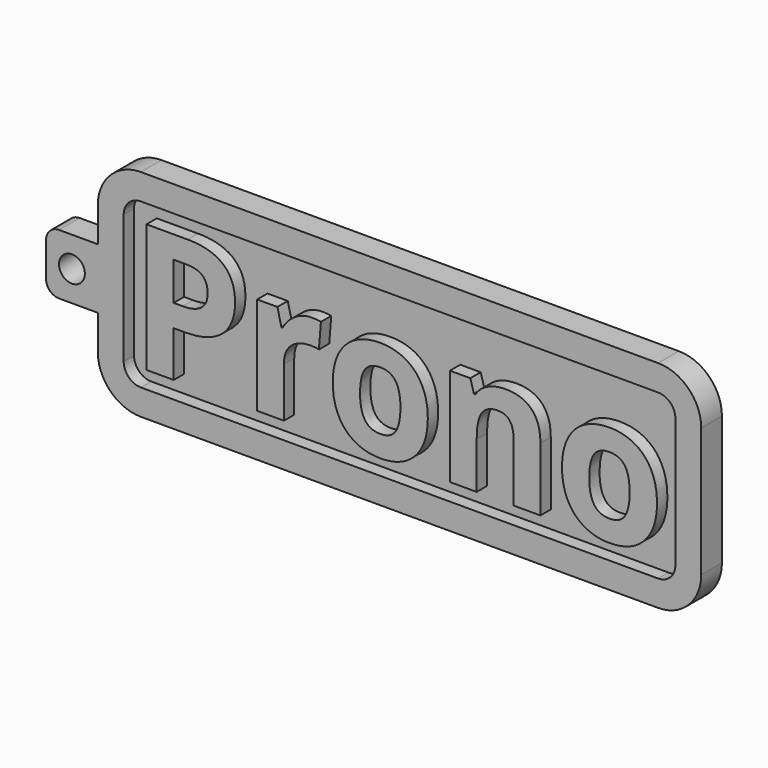
from build123d import *

# Parameters (mm, degrees)
F0_W         = 70
F0_H         = 25
F1_DEPTH     = 3
F2_R         = 5
F4_DEPTH     = 1.5
F5_TEXT_SIZE = 20.8333333333
F6_DEPTH     = 1.5
F7_R         = 1.5
F8_DEPTH     = 3
F9_R         = 1.5


# Not quite as in the source:
# - Text() gives the source's letters only with a copy of the font that has no kerning and outlines rounded to 1/6400 em; it was checked with that copy


with BuildPart() as f1:
    # F0 (on Front) → F1 (new body)
    with BuildSketch(Plane.XZ):
        Rectangle(F0_W, F0_H)
    extrude(amount=-F1_DEPTH)

    # F2
    f2_edges = [f1.edges().sort_by_distance(p)[0] for p in [
        (-35, 1.5, 12.5),
        (35, 1.5, 12.5),
        (35, 1.5, -12.5),
        (-35, 1.5, -12.5),
    ]]
    fillet(f2_edges, radius=F2_R)

    # F3 (on face) → F4 (cut)
    with BuildSketch(Plane.XZ):
        with BuildLine():
            Line((30, 9.5), (-30, 9.5))
            ThreePointArc((-30, 9.5), (-31.4142135624, 8.9142135624), (-32, 7.5))
            Line((-32, 7.5), (-32, -7.5))
            ThreePointArc((-32, -7.5), (-31.4142135624, -8.9142135624), (-30, -9.5))
            Line((-30, -9.5), (30, -9.5))
            ThreePointArc((30, -9.5), (31.4142135624, -8.9142135624), (32, -7.5))
            Line((32, -7.5), (32, 7.5))
            ThreePointArc((32, 7.5), (31.4142135624, 8.9142135624), (30, 9.5))
        make_face()
    extrude(amount=-F4_DEPTH, mode=Mode.SUBTRACT)

    # F5 (on face) → F6 (join)
    with BuildSketch(Plane.XZ.offset(-1.5)):
        with Locations((-31.2239583333, -7.5)):
            Text('Prono', F5_TEXT_SIZE, font='Open Sans', font_style=FontStyle.BOLD, text_align=(TextAlign.LEFT, TextAlign.BOTTOM))
    extrude(amount=F6_DEPTH)

    # F7 (on face) → F8 (join)
    with BuildSketch(Plane(origin=(0, 3, 0), x_dir=(-1, 0, 0), z_dir=(0, 1, 0))):
        Polygon((41, 3.5), (35, 3.5), (35, -3.5), (41, -3.5), (41, 0), align=None)
        with Locations((38, 0)):
            Circle(F7_R, mode=Mode.SUBTRACT)
    extrude(amount=-F8_DEPTH)

    # F9
    f9_edges = [f1.edges().sort_by_distance(p)[0] for p in [
        (-41, 1.5, 3.5),
        (-41, 1.5, -3.5),
    ]]
    fillet(f9_edges, radius=F9_R)


solid = f1.part
